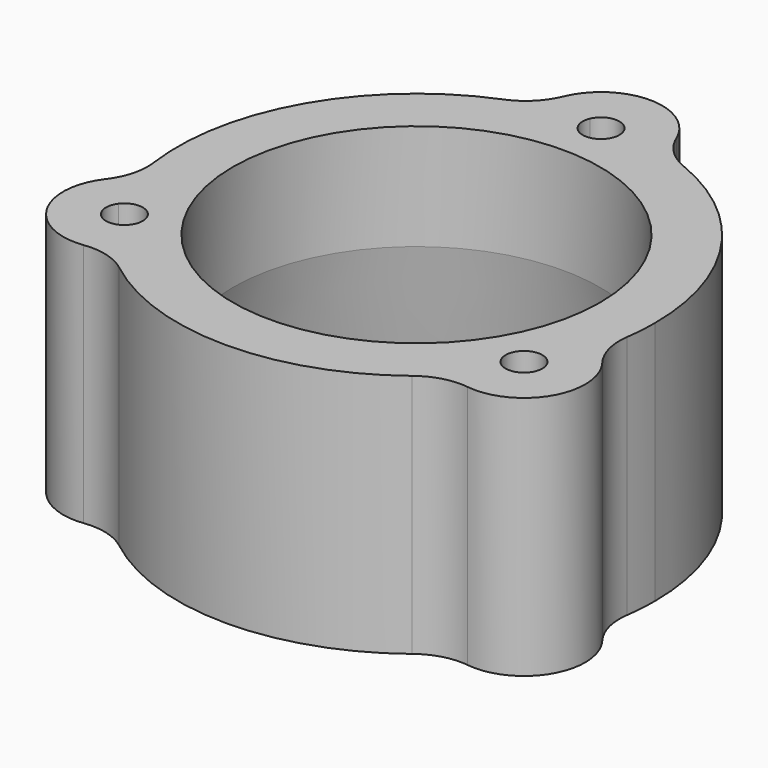
from build123d import *

# Parameters (mm, degrees)
F0_R     = 19.05
F1_DEPTH = 25.4
F2_R     = 6.35
F3_SIZE2 = 14.4050558218
F3_SIZE  = 2.54


with BuildPart() as f1:
    # F0 (on Top) → F1 (new body)
    with BuildSketch(Plane.XY):
        with BuildLine():
            ThreePointArc((23.7041161885, -4.5293078328), (24.3480999851, -1.3231236326), (24.564016243, 1.9399596371))
            ThreePointArc((24.564016243, 1.9399596371), (19.4276047684, 17.0404145143), (6.149016243, 25.8770172048))
            ThreePointArc((6.149016243, 25.8770172048), (3.8641251316, 26.3690430158), (1.5430253852, 26.6434747131))
            ThreePointArc((1.5430253852, 26.6434747131), (1.6633341365, 26.2686085633), (1.704016243, 25.8770172048))
            ThreePointArc((1.704016243, 25.8770172048), (-0.5925751155, 24.0126993113), (-1.9449928991, 26.6434747131))
            ThreePointArc((-1.9449928991, 26.6434747131), (-4.2660926456, 26.3690430158), (-6.550983757, 25.8770172048))
            ThreePointArc((-6.550983757, 25.8770172048), (-21.6481028817, 14.3224596371), (-24.1060837025, -4.5293078328))
            ThreePointArc((-24.1060837025, -4.5293078328), (-23.3897449984, -6.7540944856), (-22.4668599467, -8.9014416794))
            ThreePointArc((-22.4668599467, -8.9014416794), (-20.3380528201, -8.218226811), (-19.0260837025, -10.0285691468))
            ThreePointArc((-19.0260837025, -10.0285691468), (-19.5123327253, -11.2998561579), (-20.7228508045, -11.9221541225))
            ThreePointArc((-20.7228508045, -11.9221541225), (-19.3246361098, -13.795069619), (-17.7560837025, -15.5278304608))
            ThreePointArc((-17.7560837025, -15.5278304608), (-0.200983757, -22.8250403629), (17.3541161885, -15.5278304608))
            ThreePointArc((17.3541161885, -15.5278304608), (18.9226685958, -13.795069619), (20.3208832906, -11.9221541225))
            ThreePointArc((20.3208832906, -11.9221541225), (18.8793377943, -9.0760691468), (22.0648924327, -8.9014416794))
            ThreePointArc((22.0648924327, -8.9014416794), (22.9877774845, -6.7540944856), (23.7041161885, -4.5293078328))
        make_face()
        with Locations((-0.200983757, 1.9399596371)):
            Circle(F0_R, mode=Mode.SUBTRACT)
        with BuildLine():
            ThreePointArc((1.5430253852, 26.6434747131), (3.8641251316, 26.3690430158), (6.149016243, 25.8770172048))
            ThreePointArc((6.149016243, 25.8770172048), (-0.200983757, 32.2270172048), (-6.550983757, 25.8770172048))
            ThreePointArc((-6.550983757, 25.8770172048), (-4.2660926456, 26.3690430158), (-1.9449928991, 26.6434747131))
            ThreePointArc((-1.9449928991, 26.6434747131), (-0.200983757, 27.7820172048), (1.5430253852, 26.6434747131))
        make_face()
        with BuildLine():
            ThreePointArc((17.3541161885, -15.5278304608), (26.0283775025, -13.2035691468), (23.7041161885, -4.5293078328))
            ThreePointArc((23.7041161885, -4.5293078328), (22.9877774845, -6.7540944856), (22.0648924327, -8.9014416794))
            ThreePointArc((22.0648924327, -8.9014416794), (22.3394585243, -9.4355382645), (22.4341161885, -10.0285691468))
            ThreePointArc((22.4341161885, -10.0285691468), (21.8004031997, -11.447320124), (20.3208832906, -11.9221541225))
            ThreePointArc((20.3208832906, -11.9221541225), (18.9226685958, -13.795069619), (17.3541161885, -15.5278304608))
        make_face()
        with BuildLine():
            ThreePointArc((-22.4668599467, -8.9014416794), (-23.3897449984, -6.7540944856), (-24.1060837025, -4.5293078328))
            ThreePointArc((-24.1060837025, -4.5293078328), (-26.4303450165, -13.2035691468), (-17.7560837025, -15.5278304608))
            ThreePointArc((-17.7560837025, -15.5278304608), (-19.3246361098, -13.795069619), (-20.7228508045, -11.9221541225))
            ThreePointArc((-20.7228508045, -11.9221541225), (-22.5808620967, -10.9810691468), (-22.4668599467, -8.9014416794))
        make_face()
    extrude(amount=F1_DEPTH)

    # F2
    f2_edges = [f1.edges().sort_by_distance(p)[0] for p in [
        (-24.106084, -4.529308, 12.7),
        (17.354116, -15.52783, 12.7),
        (6.149016, 25.877017, 12.7),
        (23.704116, -4.529308, 12.7),
        (-6.550984, 25.877017, 12.7),
        (-17.756084, -15.52783, 12.7),
    ]]
    fillet(f2_edges, radius=F2_R)

    # F3
    f3_edges = [f1.edges().sort_by_distance(p)[0] for p in [
        (-19.250984, 1.93996, 0),
    ]]
    f3_side = f1.faces().sort_by_distance((20.577327, 13.936323, 0))[0]
    chamfer(f3_edges, length=F3_SIZE, length2=F3_SIZE2, reference=f3_side)


solid = f1.part
